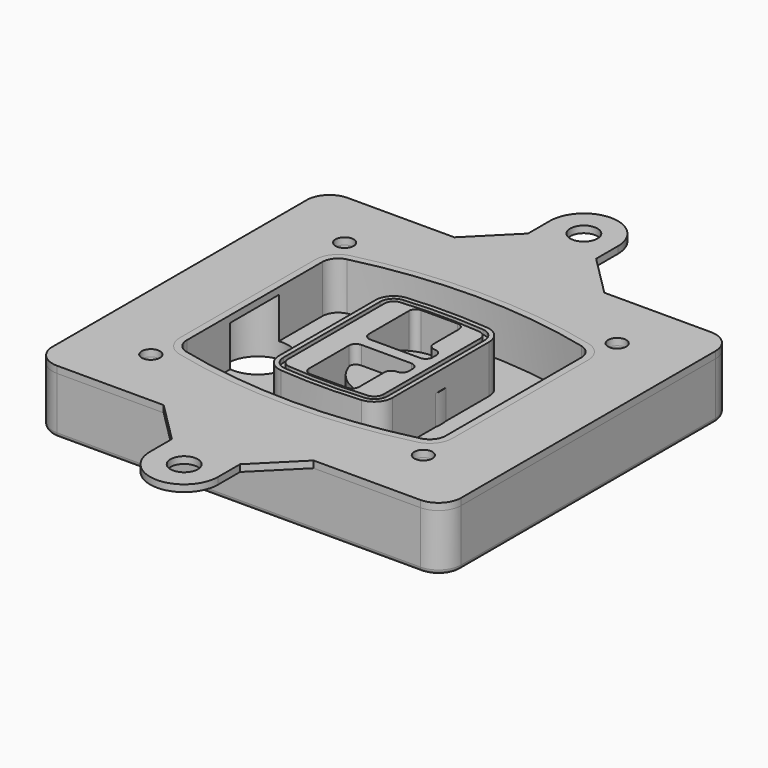
from build123d import *

# Parameters (mm, degrees)
F0_R      = 4
F1_DEPTH  = 25
F2_DEPTH  = 3
F3_DEPTH  = 18
F5_DEPTH  = 21
F6_DEPTH  = 2
F8_DEPTH  = 20
F9_DEPTH  = 16
F10_DEPTH = 25
F7_R      = 6
F7_R_2    = 4
F11_DEPTH = 6
F13_DEPTH = 9
F15_R     = 2
F16_R     = 4
F16_R_2   = 6
F17_DEPTH = 3


# Not quite as in the source:
# - a feature of the source that left no trace in its solid (it failed there, or was rolled back) is left out
# - a feature names something its author has since deleted; it is built from what else it names


with BuildPart() as f1:
    # F0 (on Top) → F1 (new body)
    with BuildSketch(Plane.XY):
        with BuildLine():
            ThreePointArc((-90, -70), (-87.0710678119, -77.0710678119), (-80, -80))
            Line((-80, -80), (80, -80))
            ThreePointArc((80, -80), (87.0710678119, -77.0710678119), (90, -70))
            Line((90, -70), (90, 70))
            ThreePointArc((90, 70), (87.0710678119, 77.0710678119), (80, 80))
            Line((80, 80), (-80, 80))
            ThreePointArc((-80, 80), (-87.0710678119, 77.0710678119), (-90, 70))
            Line((-90, 70), (-90, -70))
        make_face()
        with Locations((-60, -53.3333333333)):
            Circle(F0_R, mode=Mode.SUBTRACT)
        with Locations((60, -53.3333333333)):
            Circle(F0_R, mode=Mode.SUBTRACT)
        with Locations((-60, 53.3333333333)):
            Circle(F0_R, mode=Mode.SUBTRACT)
        with BuildLine():
            ThreePointArc((-64, 37.2990447398), (-61.0143011354, 45.9411029726), (-53.3306899286, 50.8970778549))
            ThreePointArc((-53.3306899286, 50.8970778549), (0, 57.3333333333), (53.3306899286, 50.8970778549))
            ThreePointArc((53.3306899286, 50.8970778549), (61.0143011354, 45.9411029726), (64, 37.2990447398))
            Line((64, 37.2990447398), (64, -37.2990447398))
            ThreePointArc((64, -37.2990447398), (61.0143011354, -45.9411029726), (53.3306899286, -50.8970778549))
            ThreePointArc((53.3306899286, -50.8970778549), (0, -57.3333333333), (-53.3306899286, -50.8970778549))
            ThreePointArc((-53.3306899286, -50.8970778549), (-61.0143011354, -45.9411029726), (-64, -37.2990447398))
            Line((-64, -37.2990447398), (-64, 37.2990447398))
        make_face(mode=Mode.SUBTRACT)
        with Locations((60, 53.3333333333)):
            Circle(F0_R, mode=Mode.SUBTRACT)
        with BuildLine():
            ThreePointArc((53.3306899286, 50.8970778549), (0, 57.3333333333), (-53.3306899286, 50.8970778549))
            ThreePointArc((-53.3306899286, 50.8970778549), (-61.0143011354, 45.9411029726), (-64, 37.2990447398))
            Line((-64, 37.2990447398), (-64, -37.2990447398))
            ThreePointArc((-64, -37.2990447398), (-61.0143011354, -45.9411029726), (-53.3306899286, -50.8970778549))
            ThreePointArc((-53.3306899286, -50.8970778549), (0, -57.3333333333), (53.3306899286, -50.8970778549))
            ThreePointArc((53.3306899286, -50.8970778549), (61.0143011354, -45.9411029726), (64, -37.2990447398))
            Line((64, -37.2990447398), (64, 37.2990447398))
            ThreePointArc((64, 37.2990447398), (61.0143011354, 45.9411029726), (53.3306899286, 50.8970778549))
        make_face()
        with BuildLine():
            Line((-60, -37.2990447398), (-60, 37.2990447398))
            ThreePointArc((-60, 37.2990447398), (-57.8673579538, 43.4719434775), (-52.3790642347, 47.0119255363))
            ThreePointArc((-52.3790642347, 47.0119255363), (0, 53.3333333333), (52.3790642347, 47.0119255363))
            ThreePointArc((52.3790642347, 47.0119255363), (57.8673579538, 43.4719434775), (60, 37.2990447398))
            Line((60, 37.2990447398), (60, -37.2990447398))
            ThreePointArc((60, -37.2990447398), (57.8673579538, -43.4719434775), (52.3790642347, -47.0119255363))
            ThreePointArc((52.3790642347, -47.0119255363), (0, -53.3333333333), (-52.3790642347, -47.0119255363))
            ThreePointArc((-52.3790642347, -47.0119255363), (-57.8673579538, -43.4719434775), (-60, -37.2990447398))
        make_face(mode=Mode.SUBTRACT)
        with BuildLine():
            ThreePointArc((-52.3790642347, 47.0119255363), (-57.8673579538, 43.4719434775), (-60, 37.2990447398))
            Line((-60, 37.2990447398), (-60, -37.2990447398))
            ThreePointArc((-60, -37.2990447398), (-57.8673579538, -43.4719434775), (-52.3790642347, -47.0119255363))
            ThreePointArc((-52.3790642347, -47.0119255363), (0, -53.3333333333), (52.3790642347, -47.0119255363))
            ThreePointArc((52.3790642347, -47.0119255363), (57.8673579538, -43.4719434775), (60, -37.2990447398))
            Line((60, -37.2990447398), (60, 37.2990447398))
            ThreePointArc((60, 37.2990447398), (57.8673579538, 43.4719434775), (52.3790642347, 47.0119255363))
            ThreePointArc((52.3790642347, 47.0119255363), (0, 53.3333333333), (-52.3790642347, 47.0119255363))
        make_face()
        with BuildLine():
            ThreePointArc((51.6653449643, 44.0980612973), (55.5071505677, 41.6200738562), (57, 37.2990447398))
            Line((57, 37.2990447398), (57, -37.2990447398))
            ThreePointArc((57, -37.2990447398), (55.5071505677, -41.6200738562), (51.6653449643, -44.0980612973))
            ThreePointArc((51.6653449643, -44.0980612973), (0, -50.3333333333), (-51.6653449643, -44.0980612973))
            ThreePointArc((-51.6653449643, -44.0980612973), (-55.5071505677, -41.6200738562), (-57, -37.2990447398))
            Line((-57, -37.2990447398), (-57, 37.2990447398))
            ThreePointArc((-57, 37.2990447398), (-55.5071505677, 41.6200738562), (-51.6653449643, 44.0980612973))
            ThreePointArc((-51.6653449643, 44.0980612973), (0, 50.3333333333), (51.6653449643, 44.0980612973))
        make_face(mode=Mode.SUBTRACT)
        with BuildLine():
            Line((57, -37.2990447398), (57, 37.2990447398))
            ThreePointArc((57, 37.2990447398), (55.5071505677, 41.6200738562), (51.6653449643, 44.0980612973))
            ThreePointArc((51.6653449643, 44.0980612973), (0, 50.3333333333), (-51.6653449643, 44.0980612973))
            ThreePointArc((-51.6653449643, 44.0980612973), (-55.5071505677, 41.6200738562), (-57, 37.2990447398))
            Line((-57, 37.2990447398), (-57, -37.2990447398))
            ThreePointArc((-57, -37.2990447398), (-55.5071505677, -41.6200738562), (-51.6653449643, -44.0980612973))
            ThreePointArc((-51.6653449643, -44.0980612973), (0, -50.3333333333), (51.6653449643, -44.0980612973))
            ThreePointArc((51.6653449643, -44.0980612973), (55.5071505677, -41.6200738562), (57, -37.2990447398))
        make_face()
    extrude(amount=-F1_DEPTH)

    # F0 (on Top) → F2 (join)
    with BuildSketch(Plane.XY):
        with BuildLine():
            ThreePointArc((-52.3790642347, 47.0119255363), (-57.8673579538, 43.4719434775), (-60, 37.2990447398))
            Line((-60, 37.2990447398), (-60, -37.2990447398))
            ThreePointArc((-60, -37.2990447398), (-57.8673579538, -43.4719434775), (-52.3790642347, -47.0119255363))
            ThreePointArc((-52.3790642347, -47.0119255363), (0, -53.3333333333), (52.3790642347, -47.0119255363))
            ThreePointArc((52.3790642347, -47.0119255363), (57.8673579538, -43.4719434775), (60, -37.2990447398))
            Line((60, -37.2990447398), (60, 37.2990447398))
            ThreePointArc((60, 37.2990447398), (57.8673579538, 43.4719434775), (52.3790642347, 47.0119255363))
            ThreePointArc((52.3790642347, 47.0119255363), (0, 53.3333333333), (-52.3790642347, 47.0119255363))
        make_face()
        with BuildLine():
            ThreePointArc((51.6653449643, 44.0980612973), (55.5071505677, 41.6200738562), (57, 37.2990447398))
            Line((57, 37.2990447398), (57, -37.2990447398))
            ThreePointArc((57, -37.2990447398), (55.5071505677, -41.6200738562), (51.6653449643, -44.0980612973))
            ThreePointArc((51.6653449643, -44.0980612973), (0, -50.3333333333), (-51.6653449643, -44.0980612973))
            ThreePointArc((-51.6653449643, -44.0980612973), (-55.5071505677, -41.6200738562), (-57, -37.2990447398))
            Line((-57, -37.2990447398), (-57, 37.2990447398))
            ThreePointArc((-57, 37.2990447398), (-55.5071505677, 41.6200738562), (-51.6653449643, 44.0980612973))
            ThreePointArc((-51.6653449643, 44.0980612973), (0, 50.3333333333), (51.6653449643, 44.0980612973))
        make_face(mode=Mode.SUBTRACT)
    extrude(amount=F2_DEPTH)

    # F0 (on Top) → F3 (cut)
    with BuildSketch(Plane.XY):
        with BuildLine():
            Line((57, -37.2990447398), (57, 37.2990447398))
            ThreePointArc((57, 37.2990447398), (55.5071505677, 41.6200738562), (51.6653449643, 44.0980612973))
            ThreePointArc((51.6653449643, 44.0980612973), (0, 50.3333333333), (-51.6653449643, 44.0980612973))
            ThreePointArc((-51.6653449643, 44.0980612973), (-55.5071505677, 41.6200738562), (-57, 37.2990447398))
            Line((-57, 37.2990447398), (-57, -37.2990447398))
            ThreePointArc((-57, -37.2990447398), (-55.5071505677, -41.6200738562), (-51.6653449643, -44.0980612973))
            ThreePointArc((-51.6653449643, -44.0980612973), (0, -50.3333333333), (51.6653449643, -44.0980612973))
            ThreePointArc((51.6653449643, -44.0980612973), (55.5071505677, -41.6200738562), (57, -37.2990447398))
        make_face()
    extrude(amount=-F3_DEPTH, mode=Mode.SUBTRACT)

    # F4 (on face) → F5 (join, through all)
    with BuildSketch(Plane.XY.offset(3)):
        with BuildLine():
            ThreePointArc((-25, -26.587695628), (-22.8992979869, -31.9912392117), (-17.7004291845, -34.5569740744))
            ThreePointArc((-17.7004291845, -34.5569740744), (0, -35.3333333333), (17.7004291845, -34.5569740744))
            ThreePointArc((17.7004291845, -34.5569740744), (22.8992979869, -31.9912392117), (25, -26.587695628))
            Line((25, -26.587695628), (25, 26.587695628))
            ThreePointArc((25, 26.587695628), (22.8992979869, 31.9912392117), (17.7004291845, 34.5569740744))
            ThreePointArc((17.7004291845, 34.5569740744), (0, 35.3333333333), (-17.7004291845, 34.5569740744))
            ThreePointArc((-17.7004291845, 34.5569740744), (-22.8992979869, 31.9912392117), (-25, 26.587695628))
            Line((-25, 26.587695628), (-25, -26.587695628))
        make_face()
        with BuildLine():
            ThreePointArc((17.5253218884, 32.5646544628), (21.4244734902, 30.6403533158), (23, 26.587695628))
            Line((23, 26.587695628), (23, -26.587695628))
            ThreePointArc((23, -26.587695628), (21.4244734902, -30.6403533158), (17.5253218884, -32.5646544628))
            ThreePointArc((17.5253218884, -32.5646544628), (0, -33.3333333333), (-17.5253218884, -32.5646544628))
            ThreePointArc((-17.5253218884, -32.5646544628), (-21.4244734902, -30.6403533158), (-23, -26.587695628))
            Line((-23, -26.587695628), (-23, 26.587695628))
            ThreePointArc((-23, 26.587695628), (-21.4244734902, 30.6403533158), (-17.5253218884, 32.5646544628))
            ThreePointArc((-17.5253218884, 32.5646544628), (0, 33.3333333333), (17.5253218884, 32.5646544628))
        make_face(mode=Mode.SUBTRACT)
        with BuildLine():
            Line((23, -26.587695628), (23, 26.587695628))
            ThreePointArc((23, 26.587695628), (21.4244734902, 30.6403533158), (17.5253218884, 32.5646544628))
            ThreePointArc((17.5253218884, 32.5646544628), (0, 33.3333333333), (-17.5253218884, 32.5646544628))
            ThreePointArc((-17.5253218884, 32.5646544628), (-21.4244734902, 30.6403533158), (-23, 26.587695628))
            Line((-23, 26.587695628), (-23, -26.587695628))
            ThreePointArc((-23, -26.587695628), (-21.4244734902, -30.6403533158), (-17.5253218884, -32.5646544628))
            ThreePointArc((-17.5253218884, -32.5646544628), (0, -33.3333333333), (17.5253218884, -32.5646544628))
            ThreePointArc((17.5253218884, -32.5646544628), (21.4244734902, -30.6403533158), (23, -26.587695628))
        make_face()
        with BuildLine():
            ThreePointArc((17.3502145923, 30.5723348512), (19.9496489934, 29.2894674198), (21, 26.587695628))
            Line((21, 26.587695628), (21, -26.587695628))
            ThreePointArc((21, -26.587695628), (19.9496489934, -29.2894674198), (17.3502145923, -30.5723348512))
            ThreePointArc((17.3502145923, -30.5723348512), (0, -31.3333333333), (-17.3502145923, -30.5723348512))
            ThreePointArc((-17.3502145923, -30.5723348512), (-19.9496489934, -29.2894674198), (-21, -26.587695628))
            Line((-21, -26.587695628), (-21, 26.587695628))
            ThreePointArc((-21, 26.587695628), (-19.9496489934, 29.2894674198), (-17.3502145923, 30.5723348512))
            ThreePointArc((-17.3502145923, 30.5723348512), (0, 31.3333333333), (17.3502145923, 30.5723348512))
        make_face(mode=Mode.SUBTRACT)
        with BuildLine():
            Line((21, -26.587695628), (21, 26.587695628))
            ThreePointArc((21, 26.587695628), (19.9496489934, 29.2894674198), (17.3502145923, 30.5723348512))
            ThreePointArc((17.3502145923, 30.5723348512), (0, 31.3333333333), (-17.3502145923, 30.5723348512))
            ThreePointArc((-17.3502145923, 30.5723348512), (-19.9496489934, 29.2894674198), (-21, 26.587695628))
            Line((-21, 26.587695628), (-21, -26.587695628))
            ThreePointArc((-21, -26.587695628), (-19.9496489934, -29.2894674198), (-17.3502145923, -30.5723348512))
            ThreePointArc((-17.3502145923, -30.5723348512), (0, -31.3333333333), (17.3502145923, -30.5723348512))
            ThreePointArc((17.3502145923, -30.5723348512), (19.9496489934, -29.2894674198), (21, -26.587695628))
        make_face()
        with BuildLine():
            Line((-8, -2.5), (14, -2.5))
            ThreePointArc((14, -2.5), (16.1213203436, -3.3786796564), (17, -5.5))
            Line((17, -5.5), (17, -7.5))
            ThreePointArc((17, -7.5), (16.1213203436, -9.6213203436), (14, -10.5))
            ThreePointArc((14, -10.5), (11.8786796564, -11.3786796564), (11, -13.5))
            Line((11, -13.5), (11, -27.5))
            ThreePointArc((11, -27.5), (10.1213203436, -29.6213203436), (8, -30.5))
            Line((8, -30.5), (-8, -30.5))
            ThreePointArc((-8, -30.5), (-10.1213203436, -29.6213203436), (-11, -27.5))
            Line((-11, -27.5), (-11, -5.5))
            ThreePointArc((-11, -5.5), (-10.1213203436, -3.3786796564), (-8, -2.5))
        make_face(mode=Mode.SUBTRACT)
        with BuildLine():
            ThreePointArc((-8, 2.5), (-10.1213203436, 3.3786796564), (-11, 5.5))
            Line((-11, 5.5), (-11, 27.5))
            ThreePointArc((-11, 27.5), (-10.1213203436, 29.6213203436), (-8, 30.5))
            Line((-8, 30.5), (8, 30.5))
            ThreePointArc((8, 30.5), (10.1213203436, 29.6213203436), (11, 27.5))
            Line((11, 27.5), (11, 13.5))
            ThreePointArc((11, 13.5), (11.8786796564, 11.3786796564), (14, 10.5))
            ThreePointArc((14, 10.5), (16.1213203436, 9.6213203436), (17, 7.5))
            Line((17, 7.5), (17, 5.5))
            ThreePointArc((17, 5.5), (16.1213203436, 3.3786796564), (14, 2.5))
            Line((14, 2.5), (-8, 2.5))
        make_face(mode=Mode.SUBTRACT)
    extrude(amount=-F5_DEPTH)

    # F4 (on face) → F6 (cut)
    with BuildSketch(Plane.XY.offset(3)):
        with BuildLine():
            Line((23, -26.587695628), (23, 26.587695628))
            ThreePointArc((23, 26.587695628), (21.4244734902, 30.6403533158), (17.5253218884, 32.5646544628))
            ThreePointArc((17.5253218884, 32.5646544628), (0, 33.3333333333), (-17.5253218884, 32.5646544628))
            ThreePointArc((-17.5253218884, 32.5646544628), (-21.4244734902, 30.6403533158), (-23, 26.587695628))
            Line((-23, 26.587695628), (-23, -26.587695628))
            ThreePointArc((-23, -26.587695628), (-21.4244734902, -30.6403533158), (-17.5253218884, -32.5646544628))
            ThreePointArc((-17.5253218884, -32.5646544628), (0, -33.3333333333), (17.5253218884, -32.5646544628))
            ThreePointArc((17.5253218884, -32.5646544628), (21.4244734902, -30.6403533158), (23, -26.587695628))
        make_face()
        with BuildLine():
            ThreePointArc((17.3502145923, 30.5723348512), (19.9496489934, 29.2894674198), (21, 26.587695628))
            Line((21, 26.587695628), (21, -26.587695628))
            ThreePointArc((21, -26.587695628), (19.9496489934, -29.2894674198), (17.3502145923, -30.5723348512))
            ThreePointArc((17.3502145923, -30.5723348512), (0, -31.3333333333), (-17.3502145923, -30.5723348512))
            ThreePointArc((-17.3502145923, -30.5723348512), (-19.9496489934, -29.2894674198), (-21, -26.587695628))
            Line((-21, -26.587695628), (-21, 26.587695628))
            ThreePointArc((-21, 26.587695628), (-19.9496489934, 29.2894674198), (-17.3502145923, 30.5723348512))
            ThreePointArc((-17.3502145923, 30.5723348512), (0, 31.3333333333), (17.3502145923, 30.5723348512))
        make_face(mode=Mode.SUBTRACT)
    extrude(amount=-F6_DEPTH, mode=Mode.SUBTRACT)

    # F7 (on face) → F8 (join)
    with BuildSketch(Plane(origin=(0, 0, -25), x_dir=(1, 0, 0), z_dir=(0, 0, -1))):
        with BuildLine():
            ThreePointArc((-6.71157564, 0), (6.7567035675, 13.4682792075), (20.224982775, 0))
            Line((20.224982775, 0), (25.224982775, 0))
            ThreePointArc((25.224982775, 0), (6.7567035675, 18.4682792075), (-11.71157564, 0))
            Line((-11.71157564, 0), (-6.71157564, 0))
        make_face()
        with BuildLine():
            Line((-6.71157564, 0), (20.224982775, 0))
            ThreePointArc((20.224982775, 0), (6.7567035675, 13.4682792075), (-6.71157564, 0))
        make_face()
        with BuildLine():
            ThreePointArc((-6.71157564, 0), (6.7567035675, -13.4682792075), (20.224982775, 0))
            Line((20.224982775, 0), (-6.71157564, 0))
        make_face()
        with BuildLine():
            Line((25.224982775, 0), (20.224982775, 0))
            ThreePointArc((20.224982775, 0), (6.7567035675, -13.4682792075), (-6.71157564, 0))
            Line((-6.71157564, 0), (-11.71157564, 0))
            ThreePointArc((-11.71157564, 0), (6.7567035675, -18.4682792075), (25.224982775, 0))
        make_face()
    extrude(amount=-F8_DEPTH)

    # F7 (on face) → F9 (cut)
    with BuildSketch(Plane(origin=(0, 0, -25), x_dir=(1, 0, 0), z_dir=(0, 0, -1))):
        with BuildLine():
            Line((-6.71157564, 0), (20.224982775, 0))
            ThreePointArc((20.224982775, 0), (6.7567035675, 13.4682792075), (-6.71157564, 0))
        make_face()
        with BuildLine():
            ThreePointArc((-6.71157564, 0), (6.7567035675, -13.4682792075), (20.224982775, 0))
            Line((20.224982775, 0), (-6.71157564, 0))
        make_face()
    extrude(amount=-F9_DEPTH, mode=Mode.SUBTRACT)

    # F7 (on face) → F10 (cut)
    with BuildSketch(Plane(origin=(0, 0, -25), x_dir=(1, 0, 0), z_dir=(0, 0, -1))):
        with BuildLine():
            Line((-69.0318229325, 0), (-42.0952645175, 0))
            ThreePointArc((-42.0952645175, 0), (-55.563543725, 13.4682792075), (-69.0318229325, 0))
        make_face()
        with BuildLine():
            ThreePointArc((-69.0318229325, 0), (-55.563543725, -13.4682792075), (-42.0952645175, 0))
            Line((-42.0952645175, 0), (-69.0318229325, 0))
        make_face()
    extrude(amount=-F10_DEPTH, mode=Mode.SUBTRACT)

    # F7 (on face) → F11 (cut)
    with BuildSketch(Plane(origin=(0, 0, -25), x_dir=(1, 0, 0), z_dir=(0, 0, -1))):
        with Locations((60, -53.3333333333)):
            Circle(F7_R)
        with Locations((60, -53.3333333333)):
            Circle(F7_R_2, mode=Mode.SUBTRACT)
        with Locations((-60, -53.3333333333)):
            Circle(F7_R)
        with Locations((-60, -53.3333333333)):
            Circle(F7_R_2, mode=Mode.SUBTRACT)
        with Locations((-60, 53.3333333333)):
            Circle(F7_R)
        with Locations((-60, 53.3333333333)):
            Circle(F7_R_2, mode=Mode.SUBTRACT)
        with Locations((60, 53.3333333333)):
            Circle(F7_R)
        with Locations((60, 53.3333333333)):
            Circle(F7_R_2, mode=Mode.SUBTRACT)
    extrude(amount=-F11_DEPTH, mode=Mode.SUBTRACT)

    # F12 (on face) → F13 (cut, through all)
    with BuildSketch(Plane(origin=(0, 0, -9), x_dir=(1, 0, 0), z_dir=(0, 0, -1))):
        with BuildLine():
            ThreePointArc((20.224982775, 0), (20.1663399806, 1.2554664788), (19.9909222755, 2.5))
            Line((19.9909222755, 2.5), (14, 2.5))
            ThreePointArc((14, 2.5), (16.1213203436, 3.3786796564), (17, 5.5))
            Line((17, 5.5), (17, 7.5))
            ThreePointArc((17, 7.5), (16.1213203436, 9.6213203436), (14, 10.5))
            ThreePointArc((14, 10.5), (12.1627255951, 11.1284134507), (11.0951631559, 12.750384826))
            ThreePointArc((11.0951631559, 12.750384826), (11.0476113807, 12.7664660322), (11, 12.7823698976))
            Line((11, 12.7823698976), (11, -12.7823698976))
            ThreePointArc((11, -12.7823698976), (11.0476113807, -12.7664660322), (11.0951631559, -12.750384826))
            ThreePointArc((11.0951631559, -12.750384826), (12.1627255951, -11.1284134507), (14, -10.5))
            ThreePointArc((14, -10.5), (16.1213203436, -9.6213203436), (17, -7.5))
            Line((17, -7.5), (17, -5.5))
            ThreePointArc((17, -5.5), (16.1213203436, -3.3786796564), (14, -2.5))
            Line((14, -2.5), (19.9909222755, -2.5))
            ThreePointArc((19.9909222755, -2.5), (20.1663399806, -1.2554664788), (20.224982775, 0))
        make_face()
    extrude(amount=F13_DEPTH, mode=Mode.SUBTRACT)

    # F15
    f15_edges = [f1.edges().sort_by_distance(p)[0] for p in [
        (0, -80, -25),
        (-87.071068, -77.071068, -25),
        (-90, 0, -25),
        (-87.071068, 77.071068, -25),
        (87.071068, -77.071068, -25),
        (0, 80, -25),
        (90, 0, -25),
        (87.071068, 77.071068, -25),
    ]]
    fillet(f15_edges, radius=F15_R)


with BuildPart() as f17:
    # F16 (on face) → F17 (new body, through all)
    with BuildSketch(Plane.XY):
        with BuildLine():
            Line((-33, 80), (-80, 80))
            ThreePointArc((-80, 80), (-87.0710678119, 77.0710678119), (-90, 70))
            Line((-90, 70), (-90, -70))
            ThreePointArc((-90, -70), (-87.0710678119, -77.0710678119), (-80, -80))
            Line((-80, -80), (-33, -80))
            Line((-33, -80), (33, -80))
            Line((33, -80), (80, -80))
            ThreePointArc((80, -80), (87.0710678119, -77.0710678119), (90, -70))
            Line((90, -70), (90, 70))
            ThreePointArc((90, 70), (87.0710678119, 77.0710678119), (80, 80))
            Line((80, 80), (33, 80))
            Line((33, 80), (-33, 80))
        make_face()
        with Locations((-60, -53.3333333333)):
            Circle(F16_R, mode=Mode.SUBTRACT)
        with Locations((60, -53.3333333333)):
            Circle(F16_R, mode=Mode.SUBTRACT)
        with Locations((-60, 53.3333333333)):
            Circle(F16_R, mode=Mode.SUBTRACT)
        with BuildLine():
            ThreePointArc((-52.3790642347, 47.0119255363), (0, 53.3333333333), (52.3790642347, 47.0119255363))
            ThreePointArc((52.3790642347, 47.0119255363), (57.8673579538, 43.4719434775), (60, 37.2990447398))
            Line((60, 37.2990447398), (60, -37.2990447398))
            ThreePointArc((60, -37.2990447398), (57.8673579538, -43.4719434775), (52.3790642347, -47.0119255363))
            ThreePointArc((52.3790642347, -47.0119255363), (0, -53.3333333333), (-52.3790642347, -47.0119255363))
            ThreePointArc((-52.3790642347, -47.0119255363), (-57.8673579538, -43.4719434775), (-60, -37.2990447398))
            Line((-60, -37.2990447398), (-60, 37.2990447398))
            ThreePointArc((-60, 37.2990447398), (-57.8673579538, 43.4719434775), (-52.3790642347, 47.0119255363))
        make_face(mode=Mode.SUBTRACT)
        with Locations((60, 53.3333333333)):
            Circle(F16_R, mode=Mode.SUBTRACT)
        with BuildLine():
            Line((-15, 98), (-33, 80))
            Line((-33, 80), (33, 80))
            Line((33, 80), (15, 98))
            Line((15, 98), (15, 110))
            ThreePointArc((15, 110), (0, 125), (-15, 110))
            Line((-15, 110), (-15, 98))
        make_face()
        with Locations((0, 110)):
            Circle(F16_R_2, mode=Mode.SUBTRACT)
        with BuildLine():
            Line((33, -80), (-33, -80))
            Line((-33, -80), (-15, -98))
            Line((-15, -98), (-15, -110))
            ThreePointArc((-15, -110), (0, -125), (15, -110))
            Line((15, -110), (15, -98))
            Line((15, -98), (33, -80))
        make_face()
        with Locations((0, -110)):
            Circle(F16_R_2, mode=Mode.SUBTRACT)
    extrude(amount=F17_DEPTH)


solid = Compound([f1.part, f17.part])
